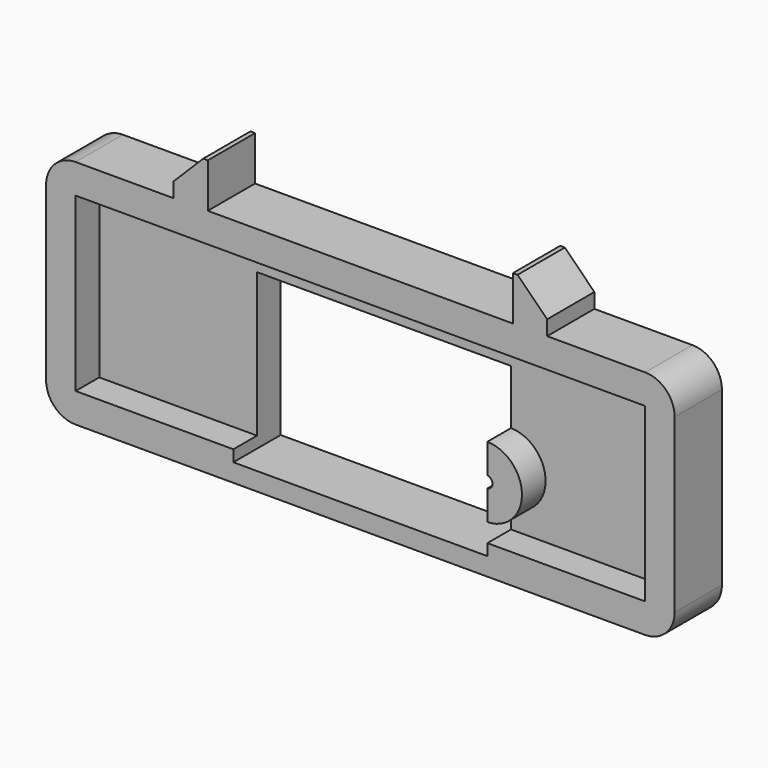
from build123d import *

# Parameters (mm, degrees)
F0_R        = 0.9849519721
F1_DEPTH    = 10
F2_T        = 5
F2_T3_DEPTH = 20
F3_SIZE     = 5
F5_DEPTH    = 25


# Not quite as in the source:
# - a shell that OpenCascade refuses in one call is made with other operations: the cavity is built on its own and cut out


with BuildPart() as f1:
    # F0 (on Front) → F1 (new body)
    with BuildSketch(Plane.XZ):
        with BuildLine():
            Line((25.823418051, 0), (0, 0))
            Line((0, 0), (-25.823418051, 0))
            Line((-25.823418051, 0), (-25.823418051, 7.5157736428))
            Line((-25.823418051, 7.5157736428), (-31.6047780216, 7.5157736428))
            Line((-31.6047780216, 7.5157736428), (-31.6047780216, 0))
            Line((-31.6047780216, 0), (-48.1885363162, 0))
            ThreePointArc((-48.1885363162, 0), (-51.7240702221, -1.4644660941), (-53.1885363162, -5))
            Line((-53.1885363162, -5), (-53.1885363162, -34.1205511987))
            ThreePointArc((-53.1885363162, -34.1205511987), (-51.7240702221, -37.6560851047), (-48.1885363162, -39.1205511987))
            Line((-48.1885363162, -39.1205511987), (0, -39.1205511987))
            Line((0, -39.1205511987), (48.1885363162, -39.1205511987))
            ThreePointArc((48.1885363162, -39.1205511987), (51.7240702221, -37.6560851047), (53.1885363162, -34.1205511987))
            Line((53.1885363162, -34.1205511987), (53.1885363162, -5))
            ThreePointArc((53.1885363162, -5), (51.7240702221, -1.4644660941), (48.1885363162, 0))
            Line((48.1885363162, 0), (31.6047780216, 0))
            Line((31.6047780216, 0), (31.6047780216, 7.5157736428))
            Line((31.6047780216, 7.5157736428), (25.823418051, 7.5157736428))
            Line((25.823418051, 7.5157736428), (25.823418051, 0))
        make_face()
        with Locations((21.3635135442, -24.997510016)):
            Circle(F0_R, mode=Mode.SUBTRACT)
    extrude(amount=F1_DEPTH)

    # F2: shell of thickness 5, made by hand


with BuildPart() as f2_core1:
    # F2_t2: copy of F1
    add(f1.part)

    # the walls: a layer under each face that stays
    f2_faces = [f2_core1.faces().sort_by_distance(p)[0] for p in [
        (39.8966571689, -5, 0),
        (20.3785615721, -5, -24.997510016),
        (53.1885363162, -5, -19.5602755994),
        (0, -5, -39.1205511987),
        (-53.1885363162, -5, -19.5602755994),
        (-39.8966571689, -5, 0),
        (-31.6047780216, -5, 3.7578868214),
        (-28.7140980363, -5, 7.5157736428),
        (-25.823418051, -5, 3.7578868214),
        (0, -5, 0),
        (25.823418051, -5, 3.7578868214),
        (28.7140980363, -5, 7.5157736428),
        (0, 0, -15.802388778),
        (31.6047780216, -5, 3.7578868214),
    ]]
    thicken(f2_faces, amount=-F2_T, mode=Mode.SUBTRACT)

    # F2_s4 → F2_t3 (cut)
    with BuildSketch(Plane.XZ.offset(-5)):
        Polygon((31.6547780216, 0.05), (31.6047780216, -5), (26.6047780216, -5), (26.6047780216, 0), align=None)
        Polygon((-31.6547780216, 0.05), (-31.6047780216, -5), (-26.6047780216, -5), (-26.6047780216, 0), align=None)
        Polygon((-25.773418051, 0.05), (-30.823418051, 0), (-30.823418051, -5), (-25.823418051, -5), align=None)
        Polygon((25.773418051, 0.05), (25.823418051, -5), (30.823418051, -5), (30.823418051, 0), align=None)
    extrude(amount=F2_T3_DEPTH, mode=Mode.SUBTRACT)


with BuildPart() as f1_1:
    add(f1.part)

    # what is left inside the walls is the cavity
    f2_cavity = [f2_core1.part.solids().sort_by_distance(p)[0] for p in [
        (0, -9.95, -24.413701),
    ]]
    add(f2_cavity, mode=Mode.SUBTRACT)

    # F3
    f3_edges = [f1_1.edges().sort_by_distance(p)[0] for p in [
        (-31.604778, -5, 7.515774),
        (31.604778, -5, 7.515774),
    ]]
    chamfer(f3_edges, length=F3_SIZE)

    # F4 (on face) → F5 (cut)
    with BuildSketch(Plane(origin=(0, 0, 0), x_dir=(-1, 0, 0), z_dir=(0, 1, 0))):
        with BuildLine():
            Line((21.4935876429, -36.0602382571), (21.4935876429, -9.7583141178))
            Line((21.4935876429, -9.7583141178), (-21.4935876429, -9.7583141178))
            Line((-21.4935876429, -9.7583141178), (-21.4935876429, -24.0211847033))
            ThreePointArc((-21.4935876429, -24.0211847033), (-20.714663158, -24.2564812961), (-20.3785615721, -24.997510016))
            ThreePointArc((-20.3785615721, -24.997510016), (-20.714663158, -25.7385387358), (-21.4935876429, -25.9738353286))
            Line((-21.4935876429, -25.9738353286), (-21.4935876429, -36.0602382571))
            Line((-21.4935876429, -36.0602382571), (21.4935876429, -36.0602382571))
        make_face()
    extrude(amount=-F5_DEPTH, mode=Mode.SUBTRACT)


solid = f1_1.part
